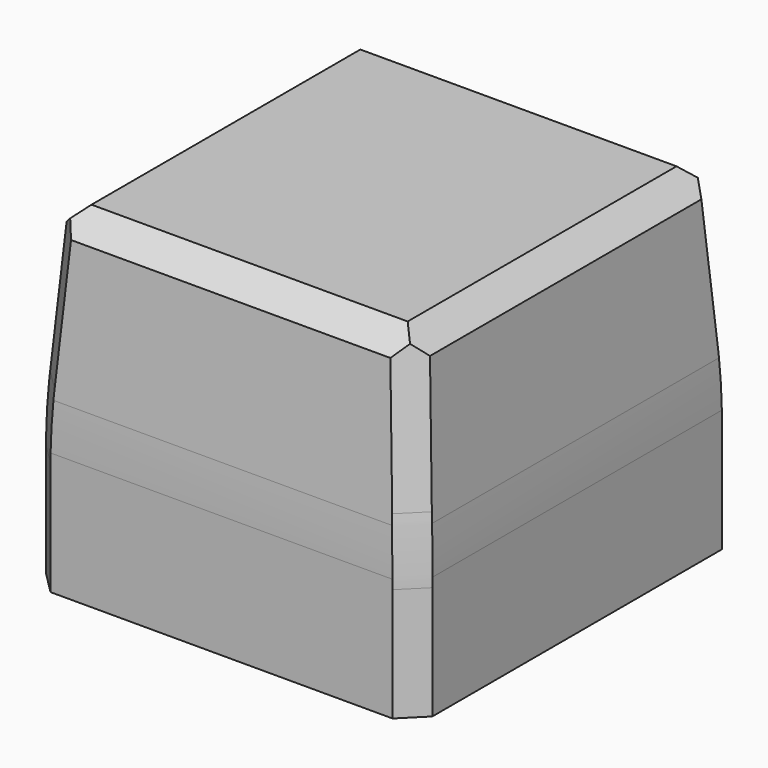
from build123d import *

# Parameters (mm, degrees)
F0_W          = 87.5
F0_H          = 92
F1_DEPTH      = 42
F1_TAPER      = 4
F1_DEPTH_BACK = 33
F5_SIZE       = 5
F6_T1_DEPTH   = 58.7168298797
F6_T3_DEPTH   = 62.7898982715
F6_T5_DEPTH   = 62.7898982715
F6_T7_DEPTH   = 62.7898982715
F6_T9_DEPTH   = 62.7898982715
F7_T1_DEPTH   = 103.6905771188
F7_T3_DEPTH   = 44.0479092504
F7_T5_DEPTH   = 44.0479092504
F7_T7_DEPTH   = 108.1905771188
F7_T9_DEPTH   = 44.0479092503
F7_T11_DEPTH  = 44.0479092503


# Not quite as in the source:
# - a fillet or chamfer that OpenCascade refuses, or shapes differently, is made with other operations: its cross-section is extruded or revolved along the edge and cut away or added


with BuildPart() as f1:
    # F0 (on Top) → F1 (new body, two sides)
    with BuildSketch(Plane.XY) as f1_sk:
        with Locations((0, -1.4119595289)):
            Rectangle(F0_W, F0_H)
    extrude(amount=F1_DEPTH, taper=F1_TAPER)
    extrude(f1_sk.sketch, amount=-F1_DEPTH_BACK)

    # F5
    f5_edges = [f1.edges().sort_by_distance(p)[0] for p in [
        (0, -44.475033, 42),
        (40.813074, -1.41196, 42),
        (0, 41.651114, 42),
        (-40.813074, -1.41196, 42),
    ]]
    chamfer(f5_edges, length=F5_SIZE)

    # F6: chamfer of 5 on 8 edges, made by hand

    # F6_s2 → F6_t1 (cut)
    with BuildSketch(Plane.XY.offset(-45.8584149398)):
        Polygon((43.75, 39.5880404711), (38.75, 44.5880404711), (43.75, 44.5880404711), align=None)
        Polygon((-43.75, 39.5880404711), (-38.75, 44.5880404711), (-43.75, 44.5880404711), align=None)
        Polygon((-38.75, -47.4119595289), (-43.75, -42.4119595289), (-43.75, -47.4119595289), align=None)
        Polygon((38.75, -47.4119595289), (43.75, -42.4119595289), (43.75, -47.4119595289), align=None)
    extrude(amount=F6_T1_DEPTH, mode=Mode.SUBTRACT)

    # F6_s4 → F6_t3 (cut)
    with BuildSketch(Plane(origin=(-1.3320626645, -1.3320626645, -19.0493835976), x_dir=(-0.7071067812, 0.7071067812, 0), z_dir=(0.0695873743, 0.0695873743, 0.9951458158))):
        Polygon((-6.1163179384, 60.6385318402), (0.9375251077, 60.6385318402), (-2.5893964153, 64.1483330365), align=None)
    extrude(amount=F6_T3_DEPTH, mode=Mode.SUBTRACT)

    # F6_s6 → F6_t5 (cut)
    with BuildSketch(Plane(origin=(1.3320626645, -1.3320626645, -19.0493835976), x_dir=(-0.7071067812, -0.7071067812, 0), z_dir=(-0.0695873743, 0.0695873743, 0.9951458158))):
        Polygon((6.1163179384, 60.6385318402), (-0.9375251077, 60.6385318402), (2.5893964153, 64.1483330365), align=None)
    extrude(amount=F6_T5_DEPTH, mode=Mode.SUBTRACT)

    # F6_s8 → F6_t7 (cut)
    with BuildSketch(Plane(origin=(-1.3183881113, 1.3183881113, -18.8538283766), x_dir=(0.7071067812, 0.7071067812, 0), z_dir=(0.0695873743, -0.0695873743, 0.9951458158))):
        Polygon((-2.934337423, 58.6514124197), (4.119505623, 58.6514124197), (0.5925841, 62.161213616), align=None)
    extrude(amount=F6_T7_DEPTH, mode=Mode.SUBTRACT)

    # F6_s10 → F6_t9 (cut)
    with BuildSketch(Plane(origin=(1.3183881113, 1.3183881113, -18.8538283766), x_dir=(0.7071067812, -0.7071067812, 0), z_dir=(-0.0695873743, -0.0695873743, 0.9951458158))):
        Polygon((2.934337423, 58.6514124197), (-4.119505623, 58.6514124197), (-0.5925841, 62.161213616), align=None)
    extrude(amount=F6_T9_DEPTH, mode=Mode.SUBTRACT)

    # F7: fillet of radius 150 on 8 edges, made by hand

    # F7_s2 → F7_t1 (cut)
    with BuildSketch(Plane.YZ.offset(-51.8452885594)):
        with BuildLine():
            ThreePointArc((-47.0465670679, 5.2253556379), (-47.3205835818, -0.0031909184), (-47.4119595289, -5.2381154238))
            Line((-47.4119595289, -5.2381154238), (-47.4119595289, 0))
            Line((-47.4119595289, 0), (-47.0465670679, 5.2253556379))
        make_face()
        with BuildLine():
            ThreePointArc((44.5880404711, -5.2381154238), (44.4966645239, -0.0031909184), (44.2226480101, 5.2253556379))
            Line((44.2226480101, 5.2253556379), (44.5880404711, 0))
            Line((44.5880404711, 0), (44.5880404711, -5.2381154238))
        make_face()
    extrude(amount=F7_T1_DEPTH, mode=Mode.SUBTRACT)

    # F7_s4 → F7_t3 (cut)
    with BuildSketch(Plane(origin=(13.7423078996, 13.7423078996, 0), x_dir=(0, 0, 1), z_dir=(-0.7071067812, -0.7071067812, 0))):
        with BuildLine():
            ThreePointArc((-7.3117239806, -60.9257058632), (0.078105005, -60.7435633688), (7.4499872987, -60.1975782307))
            Line((7.4499872987, -60.1975782307), (0.0870892603, -60.9257058632))
            Line((0.0870892603, -60.9257058632), (-7.3117239806, -60.9257058632))
        make_face()
    extrude(amount=F7_T3_DEPTH, mode=Mode.SUBTRACT)

    # F7_s6 → F7_t5 (cut)
    with BuildSketch(Plane(origin=(17.4042674285, -17.4042674285, 0), x_dir=(0, 0, 1), z_dir=(-0.7071067812, 0.7071067812, 0))):
        with BuildLine():
            ThreePointArc((7.4499872987, -60.1975782307), (0.078105005, -60.7435633688), (-7.3117239806, -60.9257058632))
            Line((-7.3117239806, -60.9257058632), (0.0870892603, -60.9257058632))
            Line((0.0870892603, -60.9257058632), (7.4499872987, -60.1975782307))
        make_face()
    extrude(amount=F7_T5_DEPTH, mode=Mode.SUBTRACT)

    # F7_s8 → F7_t7 (cut)
    with BuildSketch(Plane.XZ.offset(-52.6833290305)):
        with BuildLine():
            ThreePointArc((43.75, -5.2381154238), (43.6586240529, -0.0031909184), (43.384607539, 5.2253556379))
            Line((43.384607539, 5.2253556379), (43.75, 0))
            Line((43.75, 0), (43.75, -5.2381154238))
        make_face()
        with BuildLine():
            ThreePointArc((-43.384607539, 5.2253556379), (-43.6586240529, -0.0031909184), (-43.75, -5.2381154238))
            Line((-43.75, -5.2381154238), (-43.75, 0))
            Line((-43.75, 0), (-43.384607539, 5.2253556379))
        make_face()
    extrude(amount=F7_T7_DEPTH, mode=Mode.SUBTRACT)

    # F7_s10 → F7_t9 (cut)
    with BuildSketch(Plane(origin=(-15.1542674285, -15.1542674285, 0), x_dir=(0, 0, 1), z_dir=(0.7071067812, 0.7071067812, 0))):
        with BuildLine():
            ThreePointArc((-7.3117239809, -58.9288935479), (0.0781050046, -58.7467510535), (7.4499872984, -58.2007659154))
            Line((7.4499872984, -58.2007659154), (0.08708926, -58.9288935479))
            Line((0.08708926, -58.9288935479), (-7.3117239809, -58.9288935479))
        make_face()
    extrude(amount=F7_T9_DEPTH, mode=Mode.SUBTRACT)

    # F7_s12 → F7_t11 (cut)
    with BuildSketch(Plane(origin=(-15.9923078995, 15.9923078995, 0), x_dir=(0, 0, 1), z_dir=(0.7071067812, -0.7071067812, 0))):
        with BuildLine():
            ThreePointArc((-7.3117239809, -58.9288935479), (0.0781050046, -58.7467510535), (7.4499872984, -58.2007659154))
            Line((7.4499872984, -58.2007659154), (0.08708926, -58.9288935479))
            Line((0.08708926, -58.9288935479), (-7.3117239809, -58.9288935479))
        make_face()
    extrude(amount=F7_T11_DEPTH, mode=Mode.SUBTRACT)


solid = f1.part
